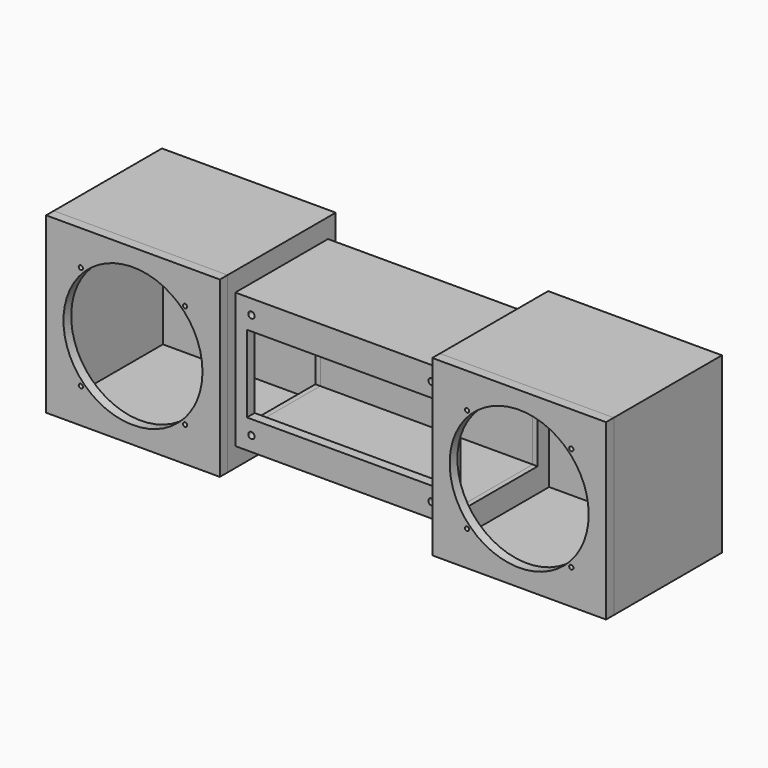
from build123d import *
from build123d import SkipClean  # not in build123d's __all__

# Parameters (mm, degrees)
F1_W      = 110
F1_H      = 70
F2_DEPTH  = 60
F4_W      = 90
F4_H      = 90
F4_R      = 1.09
F4_R_2    = 36
F5_DEPTH  = 5
F6_W      = 90
F6_H      = 90
F7_DEPTH  = 70
F8_T      = -2.54
F8_2_T    = -2.54
F9_W      = 50
F9_H      = 60
F10_DEPTH = 110
F11_W     = 50
F11_H     = 60
F12_DEPTH = 25.4
F13_W     = 50
F13_H     = 60
F14_DEPTH = 25.4
F15_W     = 98
F15_H     = 40
F15_R     = 1.65
F16_DEPTH = 25.4
F17_R     = 1.9
F17_R_2   = 1.65
F18_DEPTH = 5


# Not quite as in the source:
# - a feature names something its author has since deleted; it is built from what else it names


with BuildPart() as f2:
    # F1 (on offset) → F2 (new body)
    with BuildSketch(Plane.XZ.offset(30)):
        Rectangle(F1_W, F1_H)
    extrude(amount=-F2_DEPTH)

    # F9 (on face) → F10 (cut, through all)
    with BuildSketch(Plane.YZ.offset(55)):
        Rectangle(F9_W, F9_H)
    extrude(amount=-F10_DEPTH, mode=Mode.SUBTRACT)

    # F15 (on offset) → F16 (cut)
    with BuildSketch(Plane.XZ.offset(30)):
        Rectangle(F15_W, F15_H)
        with Locations((46.65, 27.45)):
            Circle(F15_R)
        with Locations((-46.65, 27.45)):
            Circle(F15_R)
        with Locations((-46.65, -27.45)):
            Circle(F15_R)
        with Locations((46.65, -27.45)):
            Circle(F15_R)
    extrude(amount=-F16_DEPTH, mode=Mode.SUBTRACT)

    # F17 (on face) → F18 (join)
    with BuildSketch(Plane(origin=(0, -25, 0), x_dir=(-1, 0, 0), z_dir=(0, 1, 0))):
        with Locations((-46.65, 27.45)):
            Circle(F17_R)
        with Locations((-46.65, 27.45)):
            Circle(F17_R_2, mode=Mode.SUBTRACT)
        with Locations((46.65, 27.45)):
            Circle(F17_R)
        with Locations((46.65, 27.45)):
            Circle(F17_R_2, mode=Mode.SUBTRACT)
        with Locations((46.65, -27.45)):
            Circle(F17_R)
        with Locations((46.65, -27.45)):
            Circle(F17_R_2, mode=Mode.SUBTRACT)
        with Locations((-46.65, -27.45)):
            Circle(F17_R)
        with Locations((-46.65, -27.45)):
            Circle(F17_R_2, mode=Mode.SUBTRACT)
    with SkipClean():  # cleaning this boolean's faces spoils the solid; the shape is the same uncleaned
        extrude(amount=F18_DEPTH)


with BuildPart() as f5:
    # F4 (on offset) → F5 (new body)
    with BuildSketch(Plane.XZ.offset(35)):
        with Locations((-100, 0)):
            Rectangle(F4_W, F4_H)
        with Locations((-127, -27)):
            Circle(F4_R, mode=Mode.SUBTRACT)
        with Locations((-73, -27)):
            Circle(F4_R, mode=Mode.SUBTRACT)
        with Locations((-100, 0)):
            Circle(F4_R_2, mode=Mode.SUBTRACT)
        with Locations((-127, 27)):
            Circle(F4_R, mode=Mode.SUBTRACT)
        with Locations((-73, 27)):
            Circle(F4_R, mode=Mode.SUBTRACT)
    extrude(amount=F5_DEPTH)


with BuildPart() as f5b:
    # F4 (on offset) → F5, piece 2 (new body)
    with BuildSketch(Plane.XZ.offset(35)):
        with Locations((100, 0)):
            Rectangle(F4_W, F4_H)
        with Locations((73, -27)):
            Circle(F4_R, mode=Mode.SUBTRACT)
        with Locations((127, -27)):
            Circle(F4_R, mode=Mode.SUBTRACT)
        with Locations((100, 0)):
            Circle(F4_R_2, mode=Mode.SUBTRACT)
        with Locations((73, 27)):
            Circle(F4_R, mode=Mode.SUBTRACT)
        with Locations((127, 27)):
            Circle(F4_R, mode=Mode.SUBTRACT)
    extrude(amount=F5_DEPTH)


with BuildPart() as f7:
    # F6 (on offset) → F7 (new body)
    with BuildSketch(Plane.XZ.offset(35)):
        with Locations((-100, 0)):
            Rectangle(F6_W, F6_H)
    extrude(amount=-F7_DEPTH)

    # F8
    f8_openings = [f7.faces().sort_by_distance(p)[0] for p in [
        (-100, -35, 0),
    ]]
    offset(amount=F8_T, openings=f8_openings)

    # F13 (on face) → F14 (cut)
    with BuildSketch(Plane(origin=(-57.54, 0, 0), x_dir=(0, -1, 0), z_dir=(-1, 0, 0))):
        Rectangle(F13_W, F13_H)
    extrude(amount=-F14_DEPTH, mode=Mode.SUBTRACT)


with BuildPart() as f7b:
    # F6 (on offset) → F7, piece 2 (new body)
    with BuildSketch(Plane.XZ.offset(35)):
        with Locations((100, 0)):
            Rectangle(F6_W, F6_H)
    extrude(amount=-F7_DEPTH)

    # F8#2
    f8_2_openings = [f7b.faces().sort_by_distance(p)[0] for p in [
        (100, -35, 0),
    ]]
    offset(amount=F8_2_T, openings=f8_2_openings)

    # F11 (on face) → F12 (cut)
    with BuildSketch(Plane.YZ.offset(57.54)):
        Rectangle(F11_W, F11_H)
    extrude(amount=-F12_DEPTH, mode=Mode.SUBTRACT)


solid = Compound([f2.part, f5.part, f5b.part, f7.part, f7b.part])
